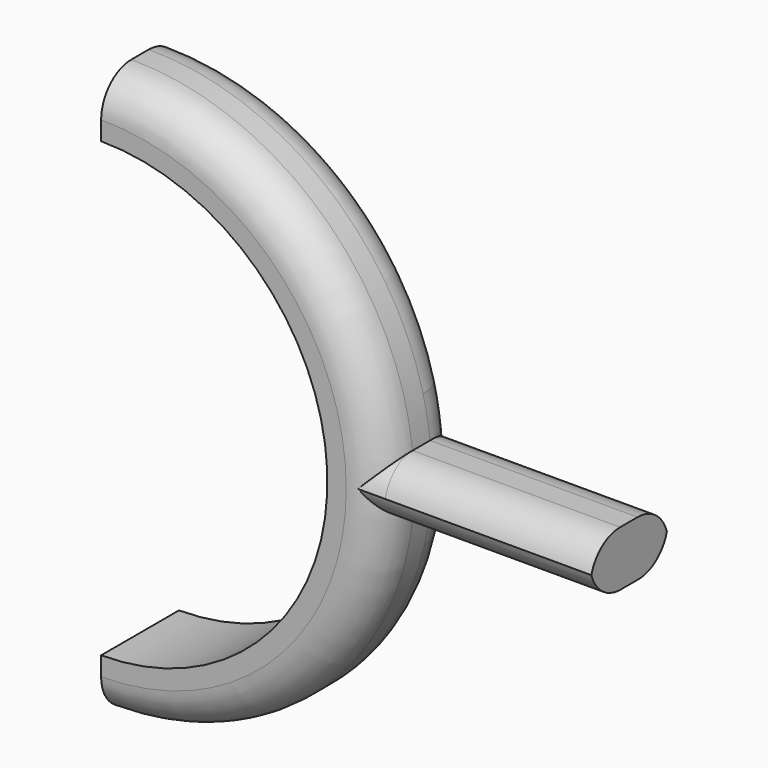
from build123d import *

# Parameters (mm, degrees)
F3_T3_DEPTH  = 53.34
F3_S4_R      = 38.080648574
F3_T5_DEPTH  = 28
F3_T8_ANGLE  = 123.2386530656
F3_T12_ANGLE = 123.2386530656
F3_T16_ANGLE = 122.1214906001
F3_T20_ANGLE = 122.1214906001
F3_T24_DEPTH = 53.34
F3_S25_R     = 38.080648574
F3_T26_DEPTH = 28
F3_T29_ANGLE = 123.2386530656
F3_T33_ANGLE = 123.2386530656
F3_T37_ANGLE = 122.1214906001
F3_T41_ANGLE = 122.1214906001
F3_T45_DEPTH = 53.3452335571
F3_S46_R     = 38.080648574
F3_T47_DEPTH = 28
F3_T50_DEPTH = 53.3452335571
F3_S51_R     = 38.080648574
F3_T52_DEPTH = 28
F3_T56_DEPTH = 53.34
F3_S57_R     = 38.080648574
F3_T58_DEPTH = 28
F3_T61_ANGLE = 122.1214906001
F3_T68_ANGLE = 123.2386530656
F3_T73_DEPTH = 53.3452335571
F3_S74_R     = 38.080648574
F3_T75_DEPTH = 28
F3_T80_DEPTH = 53.34
F3_S81_R     = 38.080648574
F3_T82_DEPTH = 28
F3_T85_ANGLE = 122.1214906001
F3_T92_ANGLE = 123.2386530656
F3_T97_DEPTH = 53.3452335571
F3_S98_R     = 38.080648574
F3_T99_DEPTH = 28


# Not quite as in the source:
# - a fillet or chamfer that OpenCascade refuses, or shapes differently, is made with other operations: its cross-section is extruded or revolved along the edge and cut away or added


with BuildPart() as f2:
    # F2: sweep along a path in F1
    with BuildLine(Plane.YZ) as f2_path:
        Line((0, 0), (13.0965914577, 0))
    # F0 (on Front) → F2 (sweep)
    with BuildSketch(Plane.XZ):
        with BuildLine():
            ThreePointArc((37.8644369888, 4.0521855022), (38.0788400668, 0.3711266463), (37.9362240869, -3.3134118136))
            Line((37.9362240869, -3.3134118136), (65.8814576441, -3.3134118136))
            Line((65.8814576441, -3.3134118136), (65.8044369888, 4.0521855022))
            Line((65.8044369888, 4.0521855022), (37.8644369888, 4.0521855022))
        make_face()
        with BuildLine():
            Line((0, -30.460648574), (0, -38.080648574))
            ThreePointArc((0, -38.080648574), (25.7289615508, -28.0741221294), (37.9362240869, -3.3134118136))
            ThreePointArc((37.9362240869, -3.3134118136), (38.0788400668, 0.3711266463), (37.8644369888, 4.0521855022))
            ThreePointArc((37.8644369888, 4.0521855022), (25.4541346716, 28.3235383373), (0, 38.080648574))
            Line((0, 38.080648574), (0, 30.460648574))
            ThreePointArc((0, 30.460648574), (30.460648574, 0), (0, -30.460648574))
        make_face()
    sweep(path=f2_path.line)

    # F3: fillet of radius 5.08 on 8 edges, made by hand


with BuildPart() as f3_tool1:
    # F3_s2 → F3_t3 (new body)
    with BuildSketch(Plane.YZ.offset(78.5044369888)):
        with BuildLine():
            ThreePointArc((0, -1.0278144978), (1.4878975516, 2.5642879506), (5.08, 4.0521855022))
            Line((5.08, 4.0521855022), (0, 4.0521855022))
            Line((0, 4.0521855022), (0, -1.0278144978))
        make_face()
    extrude(amount=-F3_T3_DEPTH)

    # F3_s4 → F3_t5 (cut, symmetric)
    with BuildSketch(Plane.XZ.offset(-2.5)):
        Circle(F3_S4_R)
    extrude(amount=F3_T5_DEPTH, both=True, mode=Mode.SUBTRACT)


with BuildPart() as f3_tool6:
    # F3_s7 → F3_t8 (revolve)
    with BuildSketch(Plane(origin=(0, 0, 0), x_dir=(0, 1, 0), z_dir=(-0.2440128994, 0, 0.969771986))):
        with BuildLine():
            ThreePointArc((0, -33.000648574), (1.4878975516, -36.5927510225), (5.08, -38.080648574))
            Line((5.08, -38.080648574), (0, -38.080648574))
            Line((0, -38.080648574), (0, -33.000648574))
        make_face()
    revolve(axis=Axis((0, 0, 0), (0, 1, 0)), revolution_arc=F3_T8_ANGLE)

    split(bisect_by=Plane.XY.offset(4.0521855022), keep=Keep.TOP)


with BuildPart() as f3_tool10:
    # F3_s11 → F3_t12 (revolve)
    with BuildSketch(Plane(origin=(0, 0, 0), x_dir=(0, 1, 0), z_dir=(-0.2440128994, 0, 0.969771986))):
        with BuildLine():
            ThreePointArc((0, -33.000648574), (1.4878975516, -36.5927510225), (5.08, -38.080648574))
            Line((5.08, -38.080648574), (0, -38.080648574))
            Line((0, -38.080648574), (0, -33.000648574))
        make_face()
    revolve(axis=Axis((0, 0, 0), (0, 1, 0)), revolution_arc=F3_T12_ANGLE)

    split(bisect_by=Plane.XY.offset(-3.3134118136), keep=Keep.BOTTOM)


with BuildPart() as f3_tool14:
    # F3_s15 → F3_t16 (revolve)
    with BuildSketch(Plane(origin=(0, 0, 0), x_dir=(0, 1, 0), z_dir=(-0.9448633995, 0, -0.3274647406))):
        with BuildLine():
            ThreePointArc((0, -33.000648574), (1.4878975516, -36.5927510225), (5.08, -38.080648574))
            Line((5.08, -38.080648574), (0, -38.080648574))
            Line((0, -38.080648574), (0, -33.000648574))
        make_face()
    revolve(axis=Axis((0, 0, 0), (0, 1, 0)), revolution_arc=F3_T16_ANGLE)

    split(bisect_by=Plane.XY.offset(4.0521855022), keep=Keep.TOP)


with BuildPart() as f3_tool18:
    # F3_s19 → F3_t20 (revolve)
    with BuildSketch(Plane(origin=(0, 0, 0), x_dir=(0, 1, 0), z_dir=(-0.9448633995, 0, -0.3274647406))):
        with BuildLine():
            ThreePointArc((0, -33.000648574), (1.4878975516, -36.5927510225), (5.08, -38.080648574))
            Line((5.08, -38.080648574), (0, -38.080648574))
            Line((0, -38.080648574), (0, -33.000648574))
        make_face()
    revolve(axis=Axis((0, 0, 0), (0, 1, 0)), revolution_arc=F3_T20_ANGLE)

    split(bisect_by=Plane.XY.offset(-3.3134118136), keep=Keep.BOTTOM)


with BuildPart() as f3_tool22:
    # F3_s23 → F3_t24 (new body)
    with BuildSketch(Plane.YZ.offset(78.5044369888)):
        with BuildLine():
            ThreePointArc((13.0965914577, -1.0278144978), (11.6086939062, 2.5642879506), (8.0165914577, 4.0521855022))
            Line((8.0165914577, 4.0521855022), (13.0965914577, 4.0521855022))
            Line((13.0965914577, 4.0521855022), (13.0965914577, -1.0278144978))
        make_face()
    extrude(amount=-F3_T24_DEPTH)

    # F3_s25 → F3_t26 (cut, symmetric)
    with BuildSketch(Plane.XZ.offset(-10.6)):
        Circle(F3_S25_R)
    extrude(amount=F3_T26_DEPTH, both=True, mode=Mode.SUBTRACT)


with BuildPart() as f3_tool27:
    # F3_s28 → F3_t29 (revolve)
    with BuildSketch(Plane(origin=(0, 0, 0), x_dir=(0, 1, 0), z_dir=(-0.9448623776, 0, 0.3274676891))):
        with BuildLine():
            ThreePointArc((8.0165914577, 38.080648574), (11.6086939062, 36.5927510225), (13.0965914577, 33.000648574))
            Line((13.0965914577, 33.000648574), (13.0965914577, 38.080648574))
            Line((13.0965914577, 38.080648574), (8.0165914577, 38.080648574))
        make_face()
    revolve(axis=Axis((0, 13.0965914577, 0), (0, -1, 0)), revolution_arc=F3_T29_ANGLE)

    split(bisect_by=Plane.XY.offset(-3.3134118136), keep=Keep.BOTTOM)


with BuildPart() as f3_tool31:
    # F3_s32 → F3_t33 (revolve)
    with BuildSketch(Plane(origin=(0, 0, 0), x_dir=(0, 1, 0), z_dir=(-0.9448623776, 0, 0.3274676891))):
        with BuildLine():
            ThreePointArc((8.0165914577, 38.080648574), (11.6086939062, 36.5927510225), (13.0965914577, 33.000648574))
            Line((13.0965914577, 33.000648574), (13.0965914577, 38.080648574))
            Line((13.0965914577, 38.080648574), (8.0165914577, 38.080648574))
        make_face()
    revolve(axis=Axis((0, 13.0965914577, 0), (0, -1, 0)), revolution_arc=F3_T33_ANGLE)

    split(bisect_by=Plane.XY.offset(4.0521855022), keep=Keep.TOP)


with BuildPart() as f3_tool35:
    # F3_s36 → F3_t37 (revolve)
    with BuildSketch(Plane(origin=(0, 0, 0), x_dir=(0, 1, 0), z_dir=(-0.2250619827, 0, -0.9743444483))):
        with BuildLine():
            ThreePointArc((13.0965914577, 33.000648574), (11.6086939062, 36.5927510225), (8.0165914577, 38.080648574))
            Line((8.0165914577, 38.080648574), (13.0965914577, 38.080648574))
            Line((13.0965914577, 38.080648574), (13.0965914577, 33.000648574))
        make_face()
    revolve(axis=Axis((0, 13.0965914577, 0), (0, -1, 0)), revolution_arc=F3_T37_ANGLE)

    split(bisect_by=Plane.XY.offset(-3.3134118136), keep=Keep.BOTTOM)


with BuildPart() as f3_tool39:
    # F3_s40 → F3_t41 (revolve)
    with BuildSketch(Plane(origin=(0, 0, 0), x_dir=(0, 1, 0), z_dir=(-0.2250619827, 0, -0.9743444483))):
        with BuildLine():
            ThreePointArc((13.0965914577, 33.000648574), (11.6086939062, 36.5927510225), (8.0165914577, 38.080648574))
            Line((8.0165914577, 38.080648574), (13.0965914577, 38.080648574))
            Line((13.0965914577, 38.080648574), (13.0965914577, 33.000648574))
        make_face()
    revolve(axis=Axis((0, 13.0965914577, 0), (0, -1, 0)), revolution_arc=F3_T41_ANGLE)

    split(bisect_by=Plane.XY.offset(4.0521855022), keep=Keep.TOP)


with BuildPart() as f3_tool43:
    # F3_s44 → F3_t45 (new body)
    with BuildSketch(Plane.YZ.offset(25.2362240869)):
        with BuildLine():
            ThreePointArc((13.0965914577, 1.7665881864), (11.6086939062, -1.8255142621), (8.0165914577, -3.3134118136))
            Line((8.0165914577, -3.3134118136), (13.0965914577, -3.3134118136))
            Line((13.0965914577, -3.3134118136), (13.0965914577, 1.7665881864))
        make_face()
    extrude(amount=F3_T45_DEPTH)

    # F3_s46 → F3_t47 (cut, symmetric)
    with BuildSketch(Plane.XZ.offset(-10.6)):
        Circle(F3_S46_R)
    extrude(amount=F3_T47_DEPTH, both=True, mode=Mode.SUBTRACT)


with BuildPart() as f3_tool48:
    # F3_s49 → F3_t50 (new body)
    with BuildSketch(Plane.YZ.offset(25.2362240869)):
        with BuildLine():
            ThreePointArc((0, 1.7665881864), (1.4878975516, -1.8255142621), (5.08, -3.3134118136))
            Line((5.08, -3.3134118136), (0, -3.3134118136))
            Line((0, -3.3134118136), (0, 1.7665881864))
        make_face()
    extrude(amount=F3_T50_DEPTH)

    # F3_s51 → F3_t52 (cut, symmetric)
    with BuildSketch(Plane.XZ.offset(-2.5)):
        Circle(F3_S51_R)
    extrude(amount=F3_T52_DEPTH, both=True, mode=Mode.SUBTRACT)


with BuildPart() as f3_tool54:
    # F3_s55 → F3_t56 (new body)
    with BuildSketch(Plane.YZ.offset(78.5044369888)):
        with BuildLine():
            ThreePointArc((0, -1.0278144978), (1.4878975516, 2.5642879506), (5.08, 4.0521855022))
            Line((5.08, 4.0521855022), (0, 4.0521855022))
            Line((0, 4.0521855022), (0, -1.0278144978))
        make_face()
    extrude(amount=-F3_T56_DEPTH)

    # F3_s57 → F3_t58 (intersect, symmetric)
    with BuildSketch(Plane.XZ.offset(-2.5)):
        Circle(F3_S57_R)
    extrude(amount=F3_T58_DEPTH, both=True, mode=Mode.INTERSECT)


with BuildPart() as f3_tool59:
    # F3_s60 → F3_t61 (revolve)
    with BuildSketch(Plane(origin=(0, 0, 0), x_dir=(0, 1, 0), z_dir=(-0.9448633995, 0, -0.3274647406))):
        with BuildLine():
            ThreePointArc((0, -33.000648574), (1.4878975516, -36.5927510225), (5.08, -38.080648574))
            Line((5.08, -38.080648574), (0, -38.080648574))
            Line((0, -38.080648574), (0, -33.000648574))
        make_face()
    revolve(axis=Axis((0, 0, 0), (0, 1, 0)), revolution_arc=F3_T61_ANGLE)

    split(bisect_by=Plane.XY.offset(-3.3134118136), keep=Keep.TOP)

    split(bisect_by=Plane.XY.offset(4.0521855022), keep=Keep.BOTTOM)


with BuildPart() as f3_tool54_1:
    add(f3_tool54.part)

    # F3_t64: intersect F3_tool59
    add(f3_tool59.part, mode=Mode.INTERSECT)


with BuildPart() as f3_tool66:
    # F3_s67 → F3_t68 (revolve)
    with BuildSketch(Plane(origin=(0, 0, 0), x_dir=(0, 1, 0), z_dir=(-0.2440128994, 0, 0.969771986))):
        with BuildLine():
            ThreePointArc((0, -33.000648574), (1.4878975516, -36.5927510225), (5.08, -38.080648574))
            Line((5.08, -38.080648574), (0, -38.080648574))
            Line((0, -38.080648574), (0, -33.000648574))
        make_face()
    revolve(axis=Axis((0, 0, 0), (0, 1, 0)), revolution_arc=F3_T68_ANGLE)

    split(bisect_by=Plane.XY.offset(-3.3134118136), keep=Keep.TOP)

    split(bisect_by=Plane.XY.offset(4.0521855022), keep=Keep.BOTTOM)


with BuildPart() as f3_tool71:
    # F3_s72 → F3_t73 (new body)
    with BuildSketch(Plane.YZ.offset(25.2362240869)):
        with BuildLine():
            ThreePointArc((0, 1.7665881864), (1.4878975516, -1.8255142621), (5.08, -3.3134118136))
            Line((5.08, -3.3134118136), (0, -3.3134118136))
            Line((0, -3.3134118136), (0, 1.7665881864))
        make_face()
    extrude(amount=F3_T73_DEPTH)

    # F3_s74 → F3_t75 (intersect, symmetric)
    with BuildSketch(Plane.XZ.offset(-2.5)):
        Circle(F3_S74_R)
    extrude(amount=F3_T75_DEPTH, both=True, mode=Mode.INTERSECT)


with BuildPart() as f3_tool66_1:
    add(f3_tool66.part)

    # F3_t76: intersect F3_tool71
    add(f3_tool71.part, mode=Mode.INTERSECT)


with BuildPart() as f3_tool78:
    # F3_s79 → F3_t80 (new body)
    with BuildSketch(Plane.YZ.offset(78.5044369888)):
        with BuildLine():
            ThreePointArc((13.0965914577, -1.0278144978), (11.6086939062, 2.5642879506), (8.0165914577, 4.0521855022))
            Line((8.0165914577, 4.0521855022), (13.0965914577, 4.0521855022))
            Line((13.0965914577, 4.0521855022), (13.0965914577, -1.0278144978))
        make_face()
    extrude(amount=-F3_T80_DEPTH)

    # F3_s81 → F3_t82 (intersect, symmetric)
    with BuildSketch(Plane.XZ.offset(-10.6)):
        Circle(F3_S81_R)
    extrude(amount=F3_T82_DEPTH, both=True, mode=Mode.INTERSECT)


with BuildPart() as f3_tool83:
    # F3_s84 → F3_t85 (revolve)
    with BuildSketch(Plane(origin=(0, 0, 0), x_dir=(0, 1, 0), z_dir=(-0.2250619827, 0, -0.9743444483))):
        with BuildLine():
            ThreePointArc((13.0965914577, 33.000648574), (11.6086939062, 36.5927510225), (8.0165914577, 38.080648574))
            Line((8.0165914577, 38.080648574), (13.0965914577, 38.080648574))
            Line((13.0965914577, 38.080648574), (13.0965914577, 33.000648574))
        make_face()
    revolve(axis=Axis((0, 13.0965914577, 0), (0, -1, 0)), revolution_arc=F3_T85_ANGLE)

    split(bisect_by=Plane.XY.offset(-3.3134118136), keep=Keep.TOP)

    split(bisect_by=Plane.XY.offset(4.0521855022), keep=Keep.BOTTOM)


with BuildPart() as f3_tool78_1:
    add(f3_tool78.part)

    # F3_t88: intersect F3_tool83
    add(f3_tool83.part, mode=Mode.INTERSECT)


with BuildPart() as f3_tool90:
    # F3_s91 → F3_t92 (revolve)
    with BuildSketch(Plane(origin=(0, 0, 0), x_dir=(0, 1, 0), z_dir=(-0.9448623776, 0, 0.3274676891))):
        with BuildLine():
            ThreePointArc((8.0165914577, 38.080648574), (11.6086939062, 36.5927510225), (13.0965914577, 33.000648574))
            Line((13.0965914577, 33.000648574), (13.0965914577, 38.080648574))
            Line((13.0965914577, 38.080648574), (8.0165914577, 38.080648574))
        make_face()
    revolve(axis=Axis((0, 13.0965914577, 0), (0, -1, 0)), revolution_arc=F3_T92_ANGLE)

    split(bisect_by=Plane.XY.offset(-3.3134118136), keep=Keep.TOP)

    split(bisect_by=Plane.XY.offset(4.0521855022), keep=Keep.BOTTOM)


with BuildPart() as f3_tool95:
    # F3_s96 → F3_t97 (new body)
    with BuildSketch(Plane.YZ.offset(25.2362240869)):
        with BuildLine():
            ThreePointArc((13.0965914577, 1.7665881864), (11.6086939062, -1.8255142621), (8.0165914577, -3.3134118136))
            Line((8.0165914577, -3.3134118136), (13.0965914577, -3.3134118136))
            Line((13.0965914577, -3.3134118136), (13.0965914577, 1.7665881864))
        make_face()
    extrude(amount=F3_T97_DEPTH)

    # F3_s98 → F3_t99 (intersect, symmetric)
    with BuildSketch(Plane.XZ.offset(-10.6)):
        Circle(F3_S98_R)
    extrude(amount=F3_T99_DEPTH, both=True, mode=Mode.INTERSECT)


with BuildPart() as f3_tool90_1:
    add(f3_tool90.part)

    # F3_t100: intersect F3_tool95
    add(f3_tool95.part, mode=Mode.INTERSECT)


with BuildPart() as f2_1:
    add(f2.part)

    # F3_t101: cut F3_tool1, F3_tool6, F3_tool10, F3_tool14, F3_tool18, F3_tool22, F3_tool27, F3_tool31, F3_tool35, F3_tool39, F3_tool43, F3_tool48, F3_tool54, F3_tool66, F3_tool78, F3_tool90
    add([f3_tool1.part, f3_tool6.part, f3_tool10.part, f3_tool14.part, f3_tool18.part, f3_tool22.part, f3_tool27.part, f3_tool31.part, f3_tool35.part, f3_tool39.part, f3_tool43.part, f3_tool48.part, f3_tool54_1.part, f3_tool66_1.part, f3_tool78_1.part, f3_tool90_1.part], mode=Mode.SUBTRACT)


solid = f2_1.part
